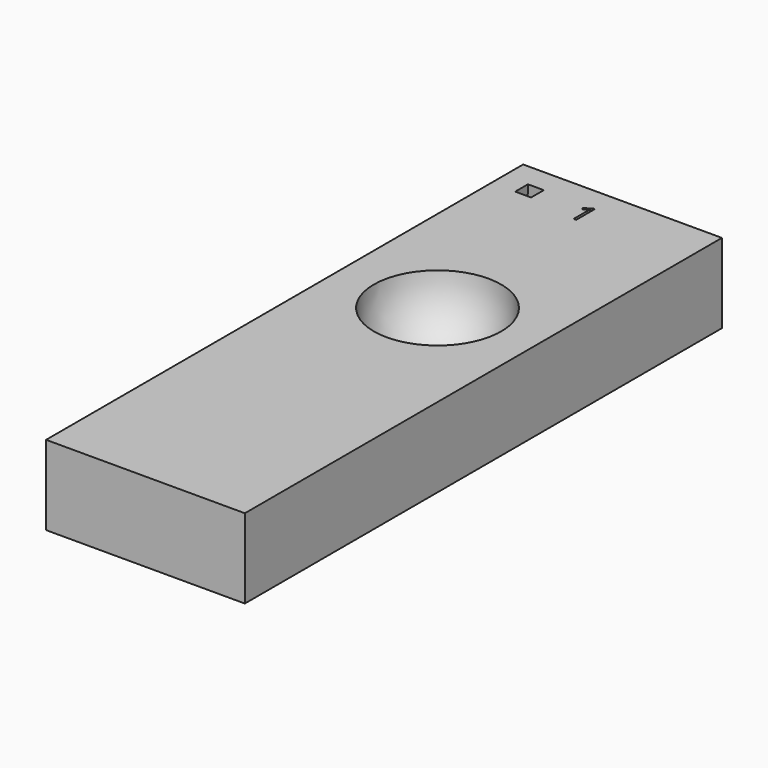
from build123d import *

# Parameters (mm, degrees)
F0_W         = 25
F0_H         = 75
F1_DEPTH     = 10
F2_W         = 2
F2_H         = 2
F3_DEPTH     = 20
F3_TAPER     = -5
F4_TEXT_SIZE = 4.0850941161
F5_DEPTH     = 20


# Not quite as in the source:
# - Text() gives the source's letters only with a copy of the font that has no kerning and outlines rounded to 1/6400 em; it was checked with that copy


with BuildPart() as f1:
    # F0 (on Top) → F1 (new body)
    with BuildSketch(Plane.XY):
        with Locations((34.8316542804, -8.4173979885)):
            Rectangle(F0_W, F0_H)
    extrude(amount=-F1_DEPTH)

    # F2 (on Top) → F3 (cut)
    with BuildSketch(Plane.XY):
        with Locations((26.3316542804, 25.0826020115)):
            Rectangle(F2_W, F2_H)
    extrude(amount=-F3_DEPTH, taper=F3_TAPER, mode=Mode.SUBTRACT)

    # F4 (on Top) → F5 (cut)
    with BuildSketch(Plane.XY):
        with Locations((32.3316542804, 23.1413342479)):
            Text('1', F4_TEXT_SIZE, font='Open Sans', text_align=(TextAlign.LEFT, TextAlign.BOTTOM))
    extrude(amount=-F5_DEPTH, mode=Mode.SUBTRACT)

    # F6 (on Front) → F7 (revolve, cut)
    with BuildSketch(Plane.XZ):
        with BuildLine():
            Line((34.8316542804, 0), (26.8316542804, 0))
            ThreePointArc((26.8316542804, 0), (29.1748000309, -5.6568542495), (34.8316542804, -8))
            Line((34.8316542804, -8), (34.8316542804, 0))
        make_face()
    revolve(axis=Axis((34.8316542804, 0, -4.9024792388), (0, 0, -1)), mode=Mode.SUBTRACT)


solid = f1.part
